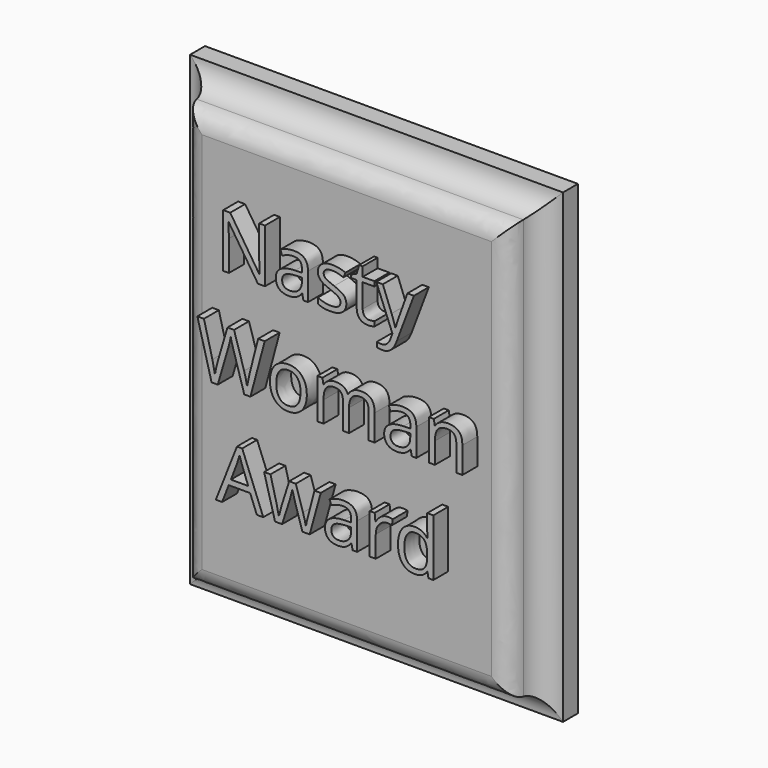
from build123d import *

# Parameters (mm, degrees)
F0_W         = 101.6
F0_H         = 127
F1_DEPTH     = 15.24
F2_W         = 101.6
F2_H         = 127
F2_W_2       = 88.9
F2_H_2       = 114.3
F3_DEPTH     = 10.16
F4_R         = 6.34999
F5_R         = 5.08
F6_TEXT_SIZE = 20.4197793364
F7_DEPTH     = 5.08


# Not quite as in the source:
# - a fillet or chamfer is up to 0.001 mm smaller than in the source, because OpenCascade refuses the exact size
# - Text() gives the source's letters only with a copy of the font that has no kerning and outlines rounded to 1/6400 em; it was checked with that copy


with BuildPart() as f1:
    # F0 (on Front) → F1 (new body)
    with BuildSketch(Plane.XZ):
        with Locations((-50.8, 63.5)):
            Rectangle(F0_W, F0_H)
    extrude(amount=F1_DEPTH)

    # F2 (on face) → F3 (cut)
    with BuildSketch(Plane.XZ.offset(15.24)):
        with Locations((-50.8, 63.5)):
            Rectangle(F2_W, F2_H)
        with Locations((-50.8, 63.5)):
            Rectangle(F2_W_2, F2_H_2, mode=Mode.SUBTRACT)
    extrude(amount=-F3_DEPTH, mode=Mode.SUBTRACT)

    # F4 (radius 6.35 in the source; OpenCascade refuses exactly that, so slightly less here)
    f4_edges = [f1.edges().sort_by_distance(p)[0] for p in [
        (-50.8, -5.08, 120.65),
        (-6.35, -5.08, 63.5),
        (-95.25, -5.08, 63.5),
        (-50.8, -5.08, 6.35),
    ]]
    fillet(f4_edges, radius=F4_R)

    # F5
    f5_edges = [f1.edges().sort_by_distance(p)[0] for p in [
        (-6.35, -15.24, 63.5),
        (-50.8, -15.24, 6.35),
        (-95.25, -15.24, 63.5),
        (-50.8, -15.24, 120.65),
    ]]
    fillet(f5_edges, radius=F5_R)

    # F6 (on face) → F7 (join)
    with BuildSketch(Plane.XZ.offset(15.24)):
        with Locations((-82.3948226373, 88.2385335521)):
            Text('Nasty', F6_TEXT_SIZE, font='Open Sans', text_align=(TextAlign.LEFT, TextAlign.BOTTOM))
        with Locations((-87.7007746743, 60.4676336545)):
            Text('Woman', F6_TEXT_SIZE, font='Open Sans', text_align=(TextAlign.LEFT, TextAlign.BOTTOM))
        with Locations((-82.3948226373, 32.696733757)):
            Text('Award', F6_TEXT_SIZE, font='Open Sans', text_align=(TextAlign.LEFT, TextAlign.BOTTOM))
    extrude(amount=F7_DEPTH)


solid = f1.part
